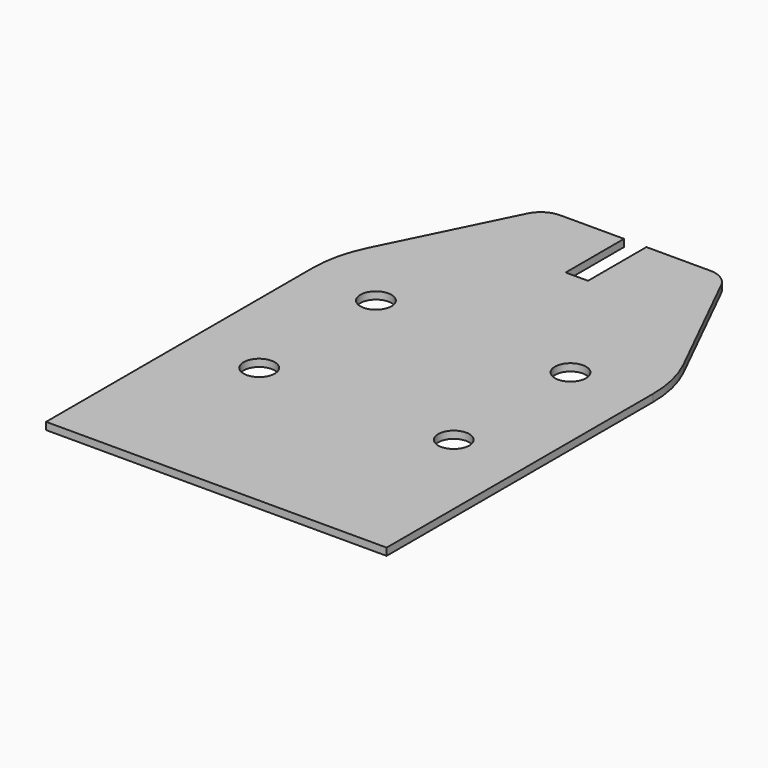
from build123d import *

# Parameters (mm, degrees)
F0_R     = 6.4
F1_DEPTH = 3


# Not quite as in the source:
# - ends of sketch curves that miss each other by under 0.0002 mm in the source are joined


with BuildPart() as f1:
    # F0 (on Top) → F1 (new body)
    with BuildSketch(Plane.XY):
        with BuildLine():
            Line((77.95862, 318.612974), (68.75862, 318.612974))
            Line((68.75862, 318.612974), (68.75862, 348.612974))
            Line((68.75862, 348.612974), (42.516137, 348.612974))
            ThreePointArc((42.516137, 348.612974), (37.2115656279, 347.0900915855), (33.5226419476, 342.9852785116))
            Line((33.5226419476, 342.9852785116), (8.391146, 292.114492))
            ThreePointArc((8.391146, 292.114492), (4.6329917176, 281.4696130444), (3.35862, 270.252967))
            Line((3.35862, 270.252967), (3.35862, 133.362974))
            Line((3.35862, 133.362974), (143.35862, 133.362974))
            Line((143.35862, 133.362974), (143.35862, 270.252967))
            ThreePointArc((143.35862, 270.252967), (142.0842482824, 281.4696130444), (138.3260940606, 292.1144920294))
            Line((138.3260940606, 292.1144920294), (113.194597, 342.985278))
            ThreePointArc((113.194597, 342.985278), (109.5056743721, 347.0900915855), (104.201103, 348.612974))
            Line((104.201103, 348.612974), (77.95862, 348.612974))
            Line((77.95862, 348.612974), (77.95862, 318.612974))
        make_face()
        with Locations((33.35862, 205.362974)):
            Circle(F0_R, mode=Mode.SUBTRACT)
        with Locations((113.35862, 205.362974)):
            Circle(F0_R, mode=Mode.SUBTRACT)
        with Locations((33.35862, 265.362974)):
            Circle(F0_R, mode=Mode.SUBTRACT)
        with Locations((113.35862, 265.362974)):
            Circle(F0_R, mode=Mode.SUBTRACT)
    extrude(amount=F1_DEPTH)


solid = f1.part
